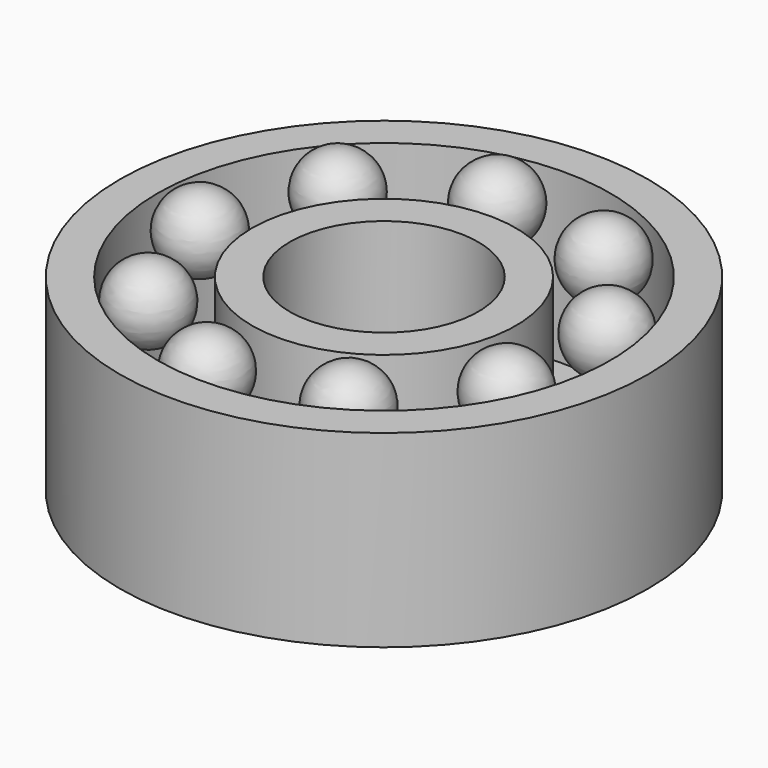
from build123d import *

# Parameters (mm, degrees)
F0_W     = 2
F0_H     = 8.9569438255
F4_COUNT = 9


with BuildPart() as f1:
    # F0 (on Front) → F1 (revolve)
    with BuildSketch(Plane.XZ):
        Polygon((-12, 8.9569438255), (-14, 8.9569438255), (-14, -1.0430561745), (-12, -1.0430561745), (-12, -1), (-12, 0), align=None)
        Polygon((-7, 0), (-12, 0), (-12, -1), (-5, -1), (-5, 0), align=None)
        with Locations((-6, 4.4784719127)):
            Rectangle(F0_W, F0_H)
    revolve(axis=Axis((0, 0, 0.9882365685), (0, 0, -1)))


with BuildPart() as f3:
    # F2 (on Front) → F3 (revolve)
    with BuildSketch(Plane.XZ):
        with BuildLine():
            Line((-9.74723602, 5.9414560129), (-9.7788500499, 9.9406480491))
            ThreePointArc((-9.7788500499, 9.9406480491), (-11.7999375123, 7.9249501678), (-9.74723602, 5.9414560129))
        make_face()
    revolve(axis=Axis((-9.7630430349, 0, 7.941052031), (0.0079048573, 0, -0.9999687561)))


with BuildPart() as f4_1:
    # F4: instance of F3
    add(f3.part.rotate(Axis((0, 0, 8.9569438255), (0, 0, -1)), 1 * 360 / F4_COUNT))


with BuildPart() as f4_2:
    # F4: instance of F3
    add(f3.part.rotate(Axis((0, 0, 8.9569438255), (0, 0, -1)), 2 * 360 / F4_COUNT))


with BuildPart() as f4_3:
    # F4: instance of F3
    add(f3.part.rotate(Axis((0, 0, 8.9569438255), (0, 0, -1)), 3 * 360 / F4_COUNT))


with BuildPart() as f4_4:
    # F4: instance of F3
    add(f3.part.rotate(Axis((0, 0, 8.9569438255), (0, 0, -1)), 4 * 360 / F4_COUNT))


with BuildPart() as f4_5:
    # F4: instance of F3
    add(f3.part.rotate(Axis((0, 0, 8.9569438255), (0, 0, -1)), 5 * 360 / F4_COUNT))


with BuildPart() as f4_6:
    # F4: instance of F3
    add(f3.part.rotate(Axis((0, 0, 8.9569438255), (0, 0, -1)), 6 * 360 / F4_COUNT))


with BuildPart() as f4_7:
    # F4: instance of F3
    add(f3.part.rotate(Axis((0, 0, 8.9569438255), (0, 0, -1)), 7 * 360 / F4_COUNT))


with BuildPart() as f4_8:
    # F4: instance of F3
    add(f3.part.rotate(Axis((0, 0, 8.9569438255), (0, 0, -1)), 8 * 360 / F4_COUNT))


solid = Compound([f1.part, f3.part, f4_1.part, f4_2.part, f4_3.part, f4_4.part, f4_5.part, f4_6.part, f4_7.part, f4_8.part])
